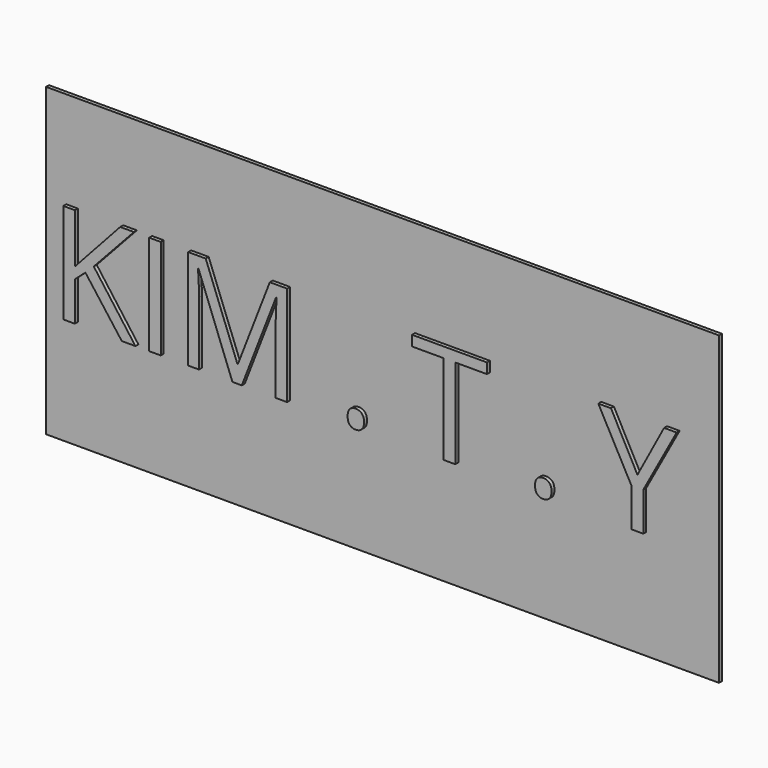
from build123d import *

# Parameters (mm, degrees)
F0_W         = 550
F0_H         = 250
F1_DEPTH     = 3
F2_TEXT_SIZE = 114.4114411441
F3_DEPTH     = 3


# Not quite as in the source:
# - Text() gives the source's letters only with a copy of the font that has no kerning and outlines rounded to 1/6400 em; it was checked with that copy


with BuildPart() as f1:
    # F0 (on Front) → F1 (new body)
    with BuildSketch(Plane.XZ):
        with Locations((275, 125)):
            Rectangle(F0_W, F0_H)
    extrude(amount=F1_DEPTH)

    # F2 (on face) → F3 (join)
    with BuildSketch(Plane.XZ.offset(3)):
        with Locations((5.2316492175, 89.2055242984)):
            Text('KIM . T . Y', F2_TEXT_SIZE, font='Open Sans', text_align=(TextAlign.LEFT, TextAlign.BOTTOM))
    extrude(amount=F3_DEPTH)


solid = f1.part
